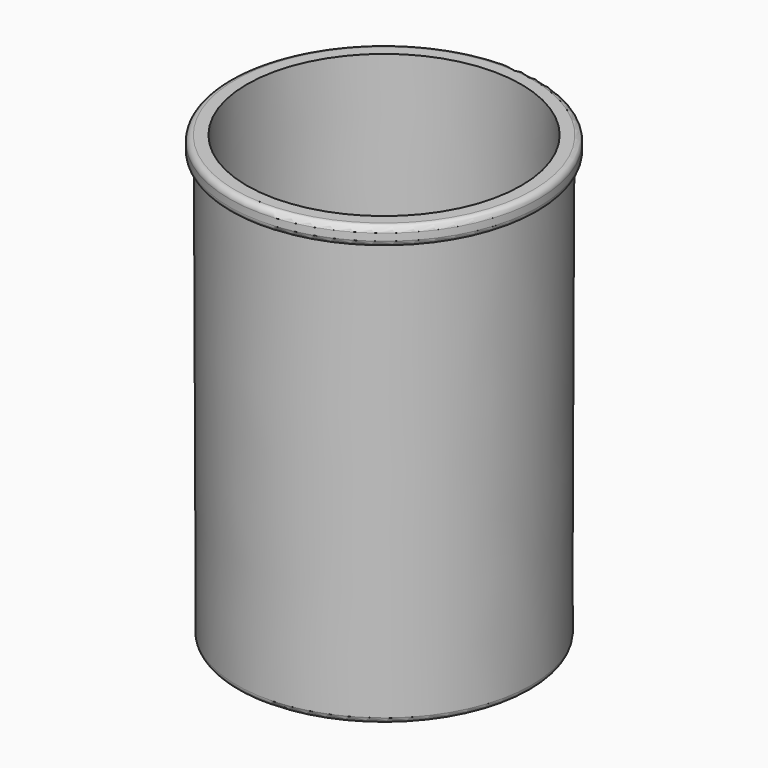
from build123d import *

# Parameters (mm, degrees)
F0_R     = 15.875
F1_DEPTH = 47.625
F1_TAPER = -0.2
F2_R     = 14.7712432865
F3_DEPTH = 45.72
F3_TAPER = 0.2
F4_R     = 16.66875
F4_R_2   = 16.0412432865
F5_DEPTH = 2.032
F6_R     = 0.635


# Not quite as in the source:
# - a fillet or chamfer that OpenCascade refuses, or shapes differently, is made with other operations: its cross-section is extruded or revolved along the edge and cut away or added


with BuildPart() as f1:
    # F0 (on Top) → F1 (new body)
    with BuildSketch(Plane.XY):
        Circle(F0_R)
    extrude(amount=F1_DEPTH, taper=F1_TAPER)

    # F2 (on face) → F3 (cut)
    with BuildSketch(Plane.XY.offset(47.625)):
        Circle(F2_R)
    extrude(amount=-F3_DEPTH, taper=F3_TAPER, mode=Mode.SUBTRACT)

    # F6
    f6_edges = [f1.edges().sort_by_distance(p)[0] for p in [
        (-15.875, 0, 0),
    ]]
    fillet(f6_edges, radius=F6_R)


with BuildPart() as f5:
    # F4 (on face) → F5 (new body)
    with BuildSketch(Plane.XY.offset(47.625)):
        Circle(F4_R)
        Circle(F4_R_2, mode=Mode.SUBTRACT)
    extrude(amount=-F5_DEPTH)

    # F7: fillet of radius 0.635 on 1 edges, made by hand

    # F7_s1 → F7_t2 (revolve, cut)
    with BuildSketch(Plane.XZ):
        with BuildLine():
            ThreePointArc((16.66875, 46.228), (16.4827628061, 45.7789871939), (16.03375, 45.593))
            Line((16.03375, 45.593), (16.66875, 45.593))
            Line((16.66875, 45.593), (16.66875, 46.228))
        make_face()
    revolve(axis=Axis((0, 0, 45.593), (0, 0, 1)), mode=Mode.SUBTRACT)

    # F8: fillet of radius 0.635 on 1 edges, made by hand

    # F8_s1 → F8_t2 (revolve, cut)
    with BuildSketch(Plane.XZ):
        with BuildLine():
            ThreePointArc((16.66875, 46.99), (16.4827628061, 47.4390128061), (16.03375, 47.625))
            Line((16.03375, 47.625), (16.66875, 47.625))
            Line((16.66875, 47.625), (16.66875, 46.99))
        make_face()
    revolve(axis=Axis((0, 0, 47.625), (0, 0, 1)), mode=Mode.SUBTRACT)


solid = Compound([f1.part, f5.part])
